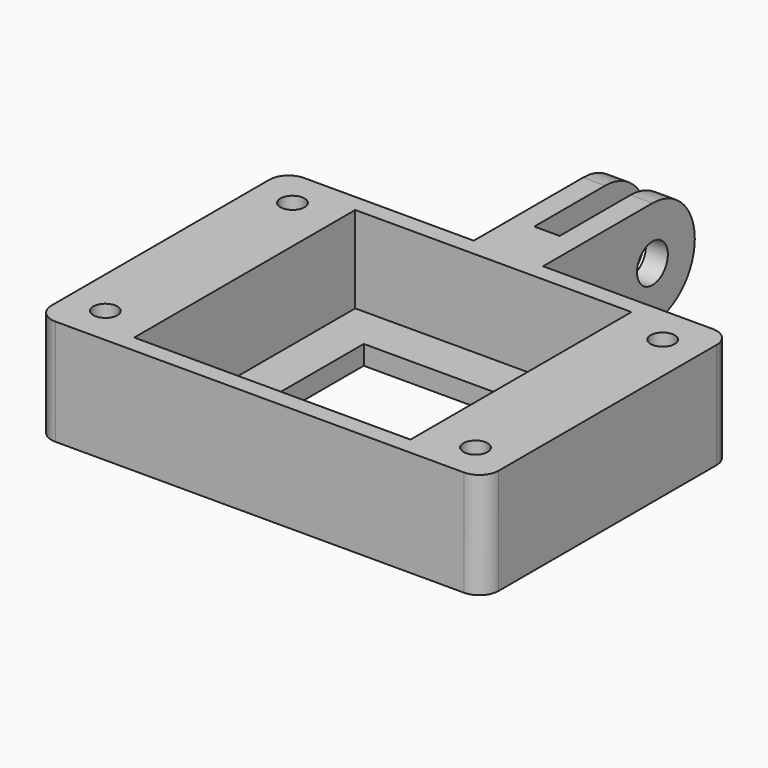
from build123d import *

# Parameters (mm, degrees)
F0_W      = 59.0042
F0_H      = 41.021
F1_DEPTH  = 13.97
F2_R      = 2.54
F3_W      = 36.449
F3_H      = 36.449
F4_DEPTH  = 11.43
F5_W      = 25.146
F5_H      = 25.146
F6_DEPTH  = 2.541
F7_R      = 1.5875
F8_DEPTH  = 12.7
F9_W      = 9.144
F9_H      = 13.97
F10_DEPTH = 25.019
F11_R     = 6.98499
F12_W     = 3.3528
F12_H     = 22.225
F13_DEPTH = 13.971
F14_R     = 2.54
F15_DEPTH = 34.0878


# Not quite as in the source:
# - a fillet or chamfer is up to 0.001 mm smaller than in the source, because OpenCascade refuses the exact size


with BuildPart() as f1:
    # F0 (on Top) → F1 (new body)
    with BuildSketch(Plane.XY):
        with Locations((4.1021, 4.8895)):
            Rectangle(F0_W, F0_H)
    extrude(amount=F1_DEPTH)

    # F2
    f2_edges = [f1.edges().sort_by_distance(p)[0] for p in [
        (-25.4, 25.4, 6.985),
        (33.6042, 25.4, 6.985),
        (33.6042, -15.621, 6.985),
        (-25.4, -15.621, 6.985),
    ]]
    fillet(f2_edges, radius=F2_R)

    # F3 (on face) → F4 (cut)
    with BuildSketch(Plane.XY.offset(13.97)):
        with Locations((3.9497, 4.8895)):
            Rectangle(F3_W, F3_H)
    extrude(amount=-F4_DEPTH, mode=Mode.SUBTRACT)

    # F5 (on face) → F6 (cut, through all)
    with BuildSketch(Plane.XY.offset(2.54)):
        with Locations((3.937, 4.9022)):
            Rectangle(F5_W, F5_H)
    extrude(amount=-F6_DEPTH, mode=Mode.SUBTRACT)

    # F7 (on face) → F8 (cut)
    with BuildSketch(Plane.XY.offset(13.97)):
        with Locations((-20.32, 20.32)):
            Circle(F7_R)
        with Locations((-20.32, -10.541)):
            Circle(F7_R)
        with Locations((28.5242, 20.32)):
            Circle(F7_R)
        with Locations((28.5242, -10.541)):
            Circle(F7_R)
    extrude(amount=-F8_DEPTH, mode=Mode.SUBTRACT)

    # F9 (on face) → F10 (join)
    with BuildSketch(Plane(origin=(0, 25.4, 0), x_dir=(-1, 0, 0), z_dir=(0, 1, 0))):
        with Locations((-4.1148, 6.985)):
            Rectangle(F9_W, F9_H)
    extrude(amount=F10_DEPTH)

    # F11 (radius 6.985 in the source; OpenCascade refuses exactly that, so slightly less here)
    f11_edges = [f1.edges().sort_by_distance(p)[0] for p in [
        (4.1148, 50.419, 13.97),
        (4.1148, 50.419, 0),
    ]]
    fillet(f11_edges, radius=F11_R)

    # F12 (on face) → F13 (cut, through all)
    with BuildSketch(Plane.XY.offset(13.97)):
        with Locations((4.1148, 42.8625)):
            Rectangle(F12_W, F12_H)
    extrude(amount=-F13_DEPTH, mode=Mode.SUBTRACT)

    # F14 (on face) → F15 (cut, through all)
    with BuildSketch(Plane.YZ.offset(8.6868)):
        with Locations((43.434, 6.985)):
            Circle(F14_R)
    extrude(amount=-F15_DEPTH, mode=Mode.SUBTRACT)


solid = f1.part
